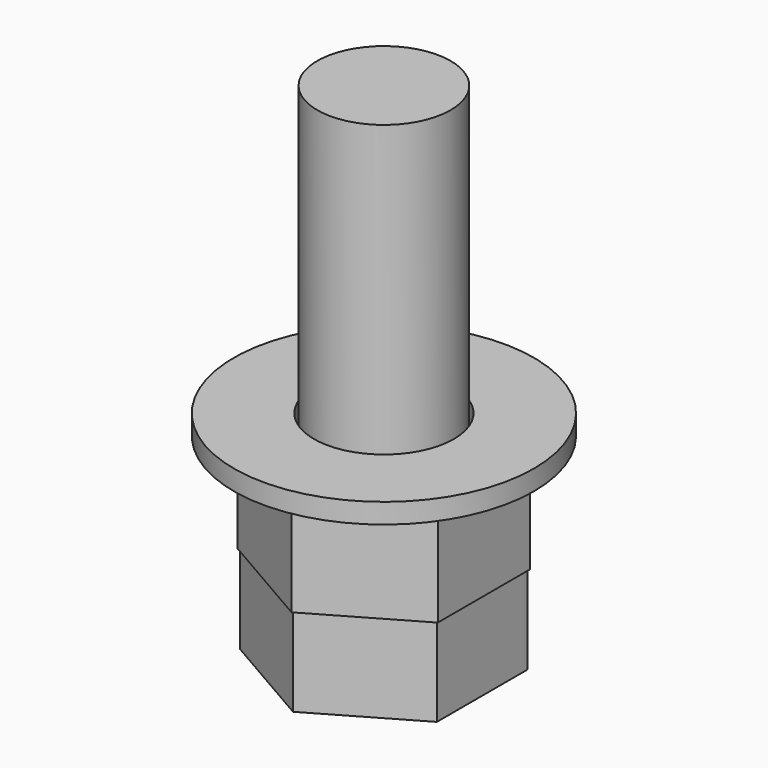
from build123d import *

# Parameters (mm, degrees)
F1_DEPTH = 5.3
F2_R     = 4
F3_DEPTH = 25
F5_DEPTH = 6.5
F6_R     = 4
F7_DEPTH = 6.5
F8_R     = 9
F8_R_2   = 4.2
F9_DEPTH = 1.2


with BuildPart() as f1:
    # F0 (on Top) → F1 (new body)
    with BuildSketch(Plane.XY):
        Polygon((0, -6.8127331764), (5.9, -3.4063665882), (5.9, 3.4063665882), (0, 6.8127331764), (-5.9, 3.4063665882), (-5.9, -3.4063665882), align=None)
    extrude(amount=F1_DEPTH)

    # F2 (on face) → F3 (join)
    with BuildSketch(Plane.XY.offset(5.3)):
        Circle(F2_R)
    extrude(amount=F3_DEPTH)


with BuildPart() as f5:
    # F4 (on face) → F5 (new body)
    with BuildSketch(Plane.XY.offset(5.3)):
        Polygon((0, -6.9282032303), (6, -3.4641016151), (6, 3.4641016151), (0, 6.9282032303), (-6, 3.4641016151), (-6, -3.4641016151), align=None)
    extrude(amount=F5_DEPTH)

    # F6 (on face) → F7 (cut)
    with BuildSketch(Plane.XY.offset(11.8)):
        Circle(F6_R)
    extrude(amount=-F7_DEPTH, mode=Mode.SUBTRACT)


with BuildPart() as f9:
    # F8 (on face) → F9 (new body)
    with BuildSketch(Plane.XY.offset(11.8)):
        Circle(F8_R)
        Circle(F8_R_2, mode=Mode.SUBTRACT)
    extrude(amount=F9_DEPTH)


solid = Compound([f1.part, f5.part, f9.part])
